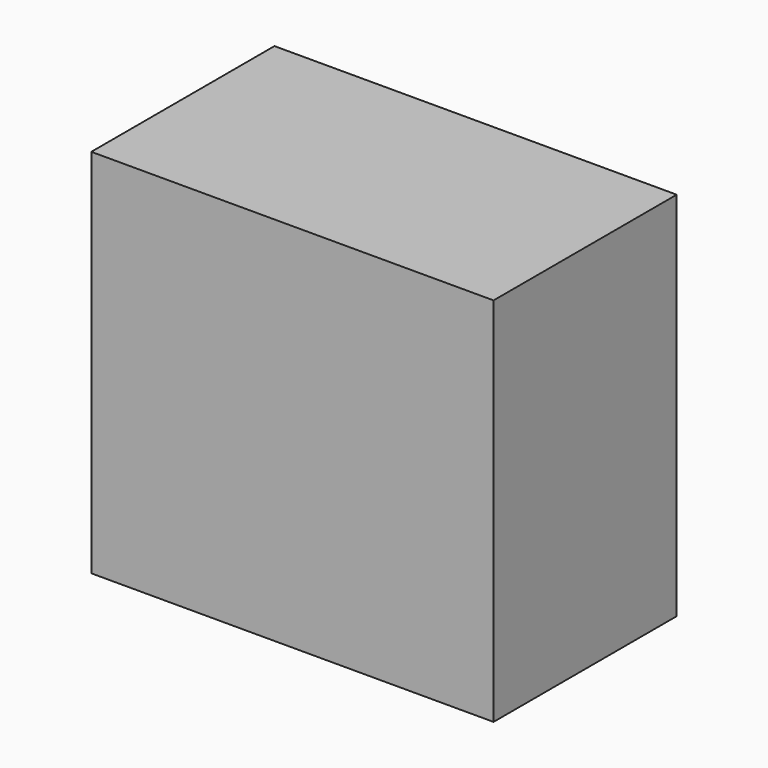
from build123d import *

# Parameters (mm, degrees)
F0_W     = 175.7008507848
F0_H     = 162.0964184403
F1_DEPTH = 100


# Not quite as in the source:
# - a feature names something its author has since deleted; it is built from what else it names


with BuildPart() as f1:
    # F0 (on Front) → F1 (new body)
    with BuildSketch(Plane.XZ):
        with Locations((-1.4757551253, -3.5817585886)):
            Rectangle(F0_W, F0_H)
    extrude(amount=-F1_DEPTH)


solid = f1.part
